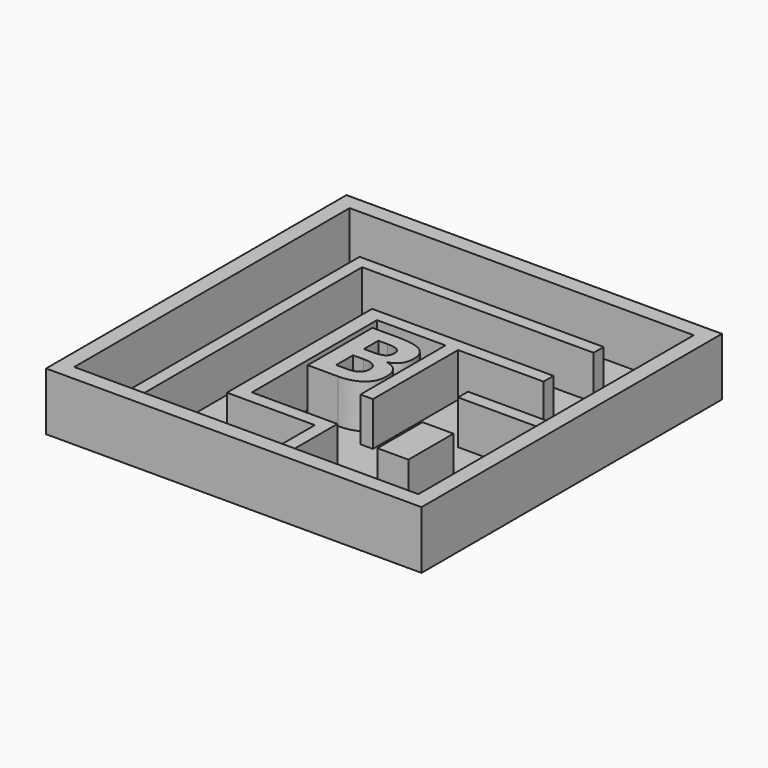
from build123d import *

# Parameters (mm, degrees)
F0_W         = 38.1
F0_H         = 38.1
F1_DEPTH     = 0.79375
F2_W         = 38.1
F2_H         = 38.1
F2_W_2       = 34.925
F2_H_2       = 34.925
F3_DEPTH     = 5.08
F4_TEXT_SIZE = 11.4919446383
F4_W         = 8.6813143664
F4_H         = 1.27
F4_W_2       = 3.1427738054
F4_H_2       = 5.715
F5_DEPTH     = 4.445
F4_R         = 1.27
F6_DEPTH     = 0.396875


# Not quite as in the source:
# - Text() gives the source's letters only with a copy of the font that has no kerning and outlines rounded to 1/6400 em; it was checked with that copy


with BuildPart() as f1:
    # F0 (on Top) → F1 (new body)
    with BuildSketch(Plane.XY):
        with Locations((-4.6593453735, 1.6864397789)):
            Rectangle(F0_W, F0_H)
    extrude(amount=F1_DEPTH)

    # F2 (on face) → F3 (join)
    with BuildSketch(Plane.XY.offset(0.79375)):
        with Locations((-4.6593453735, 1.6864397789)):
            Rectangle(F2_W, F2_H)
        with Locations((-4.6593453735, 1.6864397789)):
            Rectangle(F2_W_2, F2_H_2, mode=Mode.SUBTRACT)
    extrude(amount=F3_DEPTH)

    # F4 (on face) → F5 (join)
    with BuildSketch(Plane.XY.offset(0.79375)):
        Polygon((-17.0418453735, 14.0689397789), (-17.0418453735, -15.7760602211), (-15.7718453735, -15.7760602211), (-15.7718453735, 12.7989397789), (-9.1759614211, 12.7989397789), (7.7231546265, 12.7989397789), (7.7231546265, 14.0689397789), (-9.1759614211, 14.0689397789), (-10.6918453735, 14.0689397789), (-15.7718453735, 14.0689397789), align=None)
        Polygon((-1.769619179, -10.6960602211), (-1.769619179, -15.7760602211), (-0.499619179, -15.7760602211), (-0.499619179, -9.4260602211), (-9.1759614211, -9.4260602211), (-9.1759614211, 6.4489397789), (-2.2281597399, 6.4489397789), (-2.2281597399, -4.3460602211), (-0.9581597399, -4.3460602211), (-0.9581597399, 6.4489397789), (7.7231546265, 6.4489397789), (7.7231546265, 7.7189397789), (-9.1759614211, 7.7189397789), (-10.6918453735, 7.7189397789), (-10.6918453735, -10.6960602211), align=None)
        with Locations((-9.6648484468, -3.022468416)):
            Text('B', F4_TEXT_SIZE, font='Open Sans', font_style=FontStyle.BOLD, text_align=(TextAlign.LEFT, TextAlign.BOTTOM))
        with Locations((8.4624974433, 0.7339397789)):
            Rectangle(F4_W, F4_H)
        with Locations((6.1517677238, -7.8385602211)):
            Rectangle(F4_W_2, F4_H_2)
    extrude(amount=F5_DEPTH)

    # F4 (on face) → F6 (cut)
    with BuildSketch(Plane.XY.offset(0.79375)):
        with Locations((-19.5818453735, -11.4576322958)):
            Circle(F4_R)
        with Locations((-5.7342442573, -6.6519100219)):
            Circle(F4_R)
    extrude(amount=-F6_DEPTH, mode=Mode.SUBTRACT)


solid = f1.part
